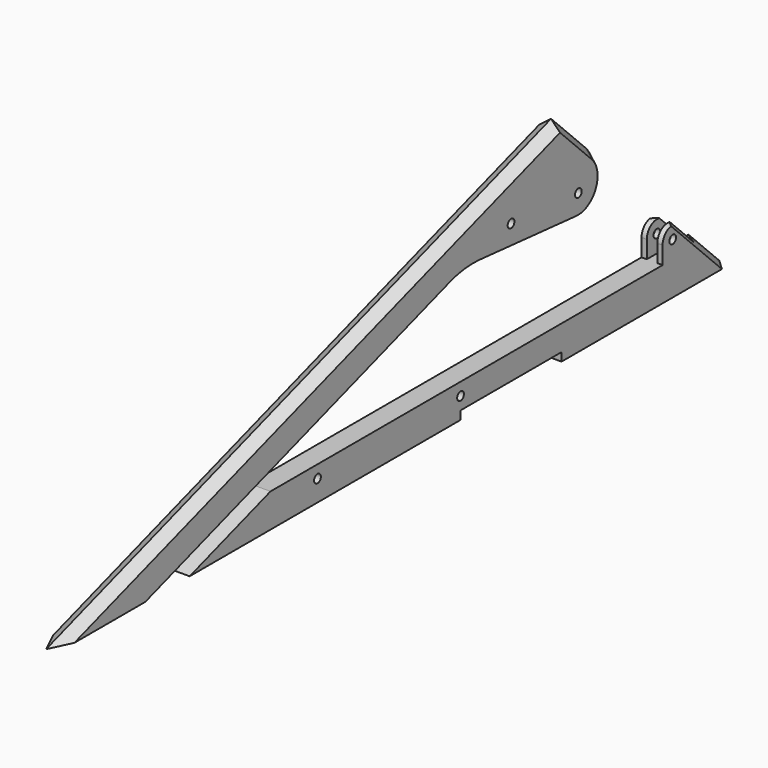
from build123d import *

# Parameters (mm, degrees)
F0_R     = 2
F1_DEPTH = 10
F2_DEPTH = 10
F3_SIZE2 = 3.3333333338
F3_SIZE  = 5
F4_SIZE2 = 3.333323
F4_SIZE  = 4.99999
F5_SIZE2 = 3.333323
F5_SIZE  = 4.99999
F6_SIZE2 = 3.333323
F6_SIZE  = 4.99999
F7_W     = 5
F7_H     = 30
F8_DEPTH = 25


# Not quite as in the source:
# - a fillet or chamfer is up to 0.001 mm smaller than in the source, because OpenCascade refuses the exact size


with BuildPart() as f1:
    # F0 (on Right) → F1 (new body)
    with BuildSketch(Plane.YZ):
        with BuildLine():
            Line((120.3614303264, 79.6385696736), (100, 100))
            Line((100, 100), (-200, 0))
            Line((-200, 0), (-136.7544467966, 0))
            Line((-136.7544467966, 0), (-46.3245553203, 30.1432971588))
            Line((-46.3245553203, 30.1432971588), (-46.9570108524, 32.0406637549))
            Line((-46.9570108524, 32.0406637549), (-27.9833448914, 38.3652190752))
            Line((-27.9833448914, 38.3652190752), (-27.3508893593, 36.4678524791))
            Line((-27.3508893593, 36.4678524791), (34.884209498, 57.2128854315))
            ThreePointArc((34.884209498, 57.2128854315), (42.8543747456, 58.9909543257), (51.0195498486, 59.1133414332))
            Line((51.0195498486, 59.1133414332), (108.4474924674, 54.0890474844))
            ThreePointArc((108.4474924674, 54.0890474844), (123.3494454141, 62.6926940297), (120.3614303264, 79.6385696736))
        make_face()
        with Locations((70, 70)):
            Circle(F0_R, mode=Mode.SUBTRACT)
        with Locations((110, 66.500453459)):
            Circle(F0_R, mode=Mode.SUBTRACT)
    extrude(amount=F1_DEPTH)

    # F3
    f3_edges = [f1.edges().sort_by_distance(p)[0] for p in [
        (10, -50, 50),
    ]]
    f3_side = f1.faces().sort_by_distance((5, -50, 50))[0]
    chamfer(f3_edges, length=F3_SIZE, length2=F3_SIZE2, reference=f3_side)

    # F4 (size 5 and 3.3333333338 in the source; OpenCascade refuses exactly that, so slightly less here)
    f4_edges = [f1.edges().sort_by_distance(p)[0] for p in [
        (0, -50, 50),
    ]]
    f4_side = f1.faces().sort_by_distance((2.5, -50, 50))[0]
    chamfer(f4_edges, length=F4_SIZE, length2=F4_SIZE2, reference=f4_side)

    # F5 (size 5 and 3.3333333338 in the source; OpenCascade refuses exactly that, so slightly less here)
    f5_edges = [f1.edges().sort_by_distance(p)[0] for p in [
        (0, 111.498327, 88.501673),
        (10, 111.498331, 88.501669),
    ]]
    f5_side = f1.faces().sort_by_distance((5, 110.824327, 89.175673))[0]
    chamfer(f5_edges, length=F5_SIZE, length2=F5_SIZE2, reference=f5_side)


with BuildPart() as f2:
    # F0 (on Right) → F2 (new body)
    with BuildSketch(Plane.YZ):
        with BuildLine():
            Line((-72.9430584958, 16), (-120.9430584958, 0))
            Line((-120.9430584958, 0), (40, 0))
            Line((40, 0), (40, 4))
            Line((40, 4), (100, 4))
            Line((100, 4), (100, 0))
            Line((100, 0), (200, 0))
            Line((200, 0), (170, 30))
            Line((170, 30), (166.5609874756, 30.3008746096))
            ThreePointArc((166.5609874756, 30.3008746096), (161.9845117734, 28.7473704419), (160.0380530191, 24.3237064211))
            Line((160.0380530191, 24.3237064211), (160.0380530191, 16))
            Line((160.0380530191, 16), (-72.9430584958, 16))
        make_face()
        with Locations((-45, 10)):
            Circle(F0_R, mode=Mode.SUBTRACT)
        with Locations((40, 10)):
            Circle(F0_R, mode=Mode.SUBTRACT)
        with Locations((166.0380530191, 24.3237064211)):
            Circle(F0_R, mode=Mode.SUBTRACT)
    extrude(amount=F2_DEPTH)

    # F6 (size 5 and 3.3333333338 in the source; OpenCascade refuses exactly that, so slightly less here)
    f6_edges = [f2.edges().sort_by_distance(p)[0] for p in [
        (0, 185, 15),
        (10, 185, 15),
    ]]
    f6_side = f2.faces().sort_by_distance((5, 185, 15))[0]
    chamfer(f6_edges, length=F6_SIZE, length2=F6_SIZE2, reference=f6_side)

    # F7 (on face) → F8 (cut)
    with BuildSketch(Plane.XY.offset(16)):
        with Locations((5, 166.5609874756)):
            Rectangle(F7_W, F7_H)
    extrude(amount=F8_DEPTH, mode=Mode.SUBTRACT)


solid = Compound([f1.part, f2.part])
